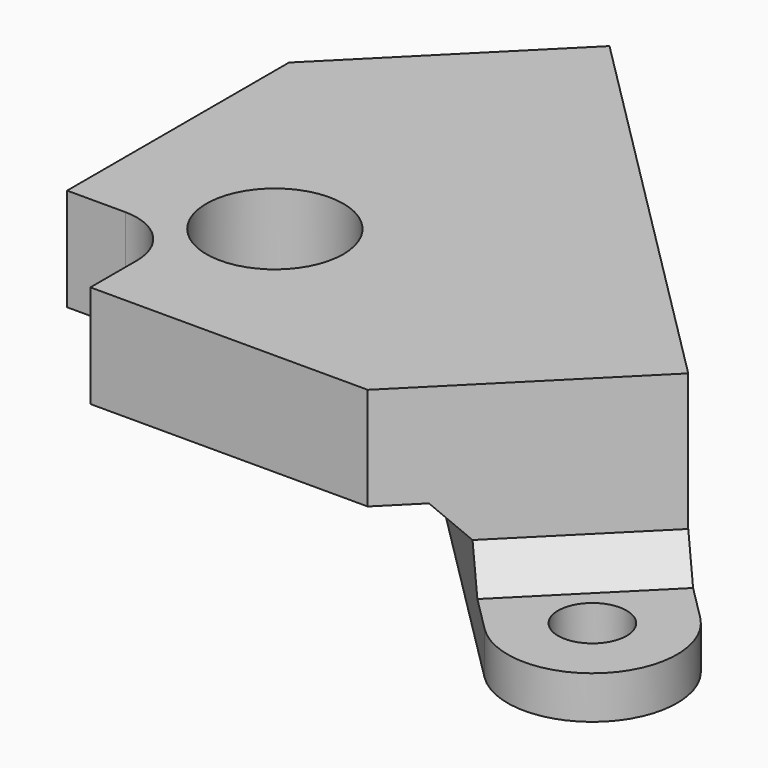
from build123d import *

# Parameters (mm, degrees)
F0_R     = 2
F1_DEPTH = 6.5
F3_DEPTH = 4
F4_R     = 4
F5_DEPTH = 6
F6_SIZE  = 1.99999


# Not quite as in the source:
# - a fillet or chamfer is up to 0.001 mm smaller than in the source, because OpenCascade refuses the exact size


with BuildPart() as f1:
    # F0 (on Top) → F1 (new body)
    with BuildSketch(Plane.XY):
        with BuildLine():
            Line((37, 7), (7, 37))
            ThreePointArc((7, 37), (0, 37), (0, 30))
            Line((0, 30), (30, 0))
            ThreePointArc((30, 0), (37, 0), (37, 7))
        make_face()
        with Locations((33.5, 3.5)):
            Circle(F0_R, mode=Mode.SUBTRACT)
        with Locations((3.5, 33.5)):
            Circle(F0_R, mode=Mode.SUBTRACT)
    extrude(amount=F1_DEPTH)

    # F2 (on face) → F3 (cut)
    with BuildSketch(Plane.XY.offset(6.5)):
        with BuildLine():
            Line((10.5, 33.5), (7, 37))
            ThreePointArc((7, 37), (0, 37), (0, 30))
            Line((0, 30), (3.5, 26.5))
            Line((3.5, 26.5), (10.5, 33.5))
        make_face()
        with BuildLine():
            Line((26.5, 3.5), (30, 0))
            ThreePointArc((30, 0), (37, 0), (37, 7))
            Line((37, 7), (33.5, 10.5))
            Line((33.5, 10.5), (26.5, 3.5))
        make_face()
    extrude(amount=-F3_DEPTH, mode=Mode.SUBTRACT)

    # F4 (on face) → F5 (join)
    with BuildSketch(Plane.XY.offset(6.5)):
        with BuildLine():
            ThreePointArc((3.5, 6.9), (5.904163056, 5.904163056), (6.9, 3.5))
            Line((6.9, 3.5), (6.9, 0.1))
            Line((6.9, 0.1), (23.1, 0.1))
            Line((23.1, 0.1), (33.5, 10.5))
            Line((33.5, 10.5), (10.5, 33.5))
            Line((10.5, 33.5), (0.1, 23.1))
            Line((0.1, 23.1), (0.1, 6.9))
            Line((0.1, 6.9), (3.5, 6.9))
        make_face()
        with Locations((9.8639610307, 9.8639610307)):
            Circle(F4_R, mode=Mode.SUBTRACT)
    extrude(amount=F5_DEPTH)

    # F6 (size 2 in the source; OpenCascade refuses exactly that, so slightly less here)
    f6_edges = [f1.edges().sort_by_distance(p)[0] for p in [
        (7, 30, 2.5),
        (15, 15, 6.5),
        (30, 7, 2.5),
    ]]
    chamfer(f6_edges, length=F6_SIZE)


solid = f1.part
